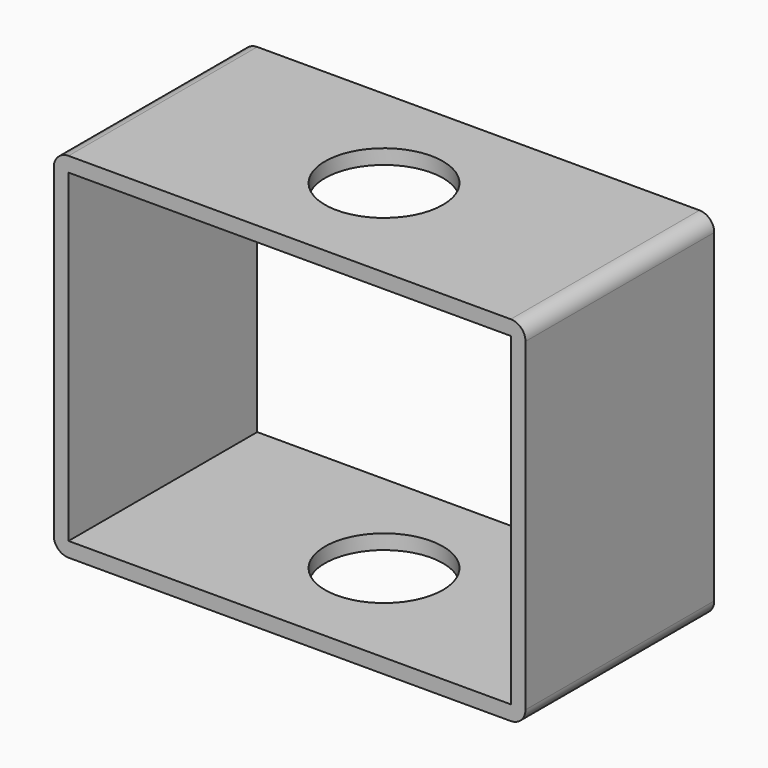
from build123d import *

# Parameters (mm, degrees)
F0_W     = 190.5
F0_H     = 139.7
F1_DEPTH = 101.6
F2_R     = 25.4
F3_DEPTH = 152.401


# Not quite as in the source:
# - ends of sketch curves that miss each other by under 0.0002 mm in the source are joined


with BuildPart() as f1:
    # F0 (on Front) → F1 (new body)
    with BuildSketch(Plane.XZ):
        with BuildLine():
            Line((-95.25, -76.2), (95.25, -76.2))
            ThreePointArc((95.25, -76.2), (99.7401280605, -74.3401280605), (101.6, -69.85))
            Line((101.6, -69.85), (101.6, 69.85))
            ThreePointArc((101.6, 69.85), (99.7401280605, 74.3401280605), (95.25, 76.2))
            Line((95.25, 76.2), (-95.25, 76.2))
            ThreePointArc((-95.25, 76.2), (-99.7401280605, 74.3401280605), (-101.6, 69.85))
            Line((-101.6, 69.85), (-101.6, -69.85))
            ThreePointArc((-101.6, -69.85), (-99.7401280605, -74.3401280605), (-95.25, -76.2))
        make_face()
        Rectangle(F0_W, F0_H, mode=Mode.SUBTRACT)
    extrude(amount=F1_DEPTH)

    # F2 (on face) → F3 (cut, through all)
    with BuildSketch(Plane.XY.offset(76.2)):
        with Locations((0, -50.8)):
            Circle(F2_R)
    extrude(amount=-F3_DEPTH, mode=Mode.SUBTRACT)


solid = f1.part
